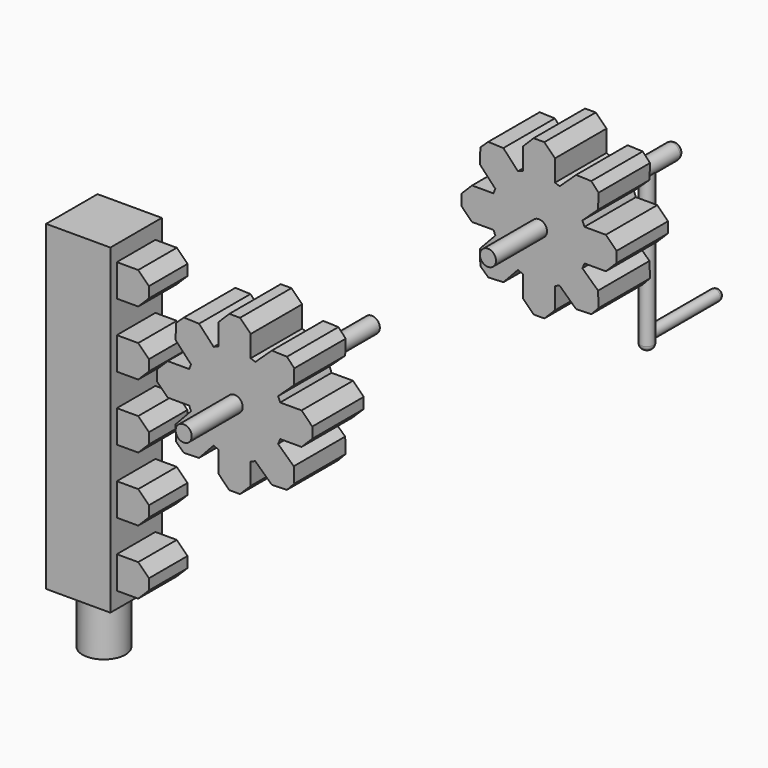
from build123d import *

# Parameters (mm, degrees)
F0_W           = 30.48
F0_H           = 30.48
F0_R           = 10.16
F1_DEPTH       = 152.4
F2_DEPTH       = 25.4
F3_W           = 22.86
F3_H           = 15.24
F4_DEPTH       = 30.48
F5_SIZE        = 5.08
F6_R           = 3.81
F7_DEPTH       = 30.48
F8_SIZE        = 5.08
F9_T1_DEPTH    = 56.6082991577
F9_T3_DEPTH    = 56.6285424882
F10_DEPTH      = 60.706
F10_DEPTH_BACK = 50.8
F13_R          = 3.1229358852
F14_DEPTH      = 76.2
F15_R          = 2.54
F17_R          = 2.667
F18_DEPTH      = 43.18
F19_R          = 2.54


# Not quite as in the source:
# - a fillet or chamfer that OpenCascade refuses, or shapes differently, is made with other operations: its cross-section is extruded or revolved along the edge and cut away or added


with BuildPart() as f1:
    # F0 (on Top) → F1 (new body)
    with BuildSketch(Plane.XY):
        Rectangle(F0_W, F0_H)
        Circle(F0_R, mode=Mode.SUBTRACT)
        Circle(F0_R)
    extrude(amount=F1_DEPTH)

    # F0 (on Top) → F2 (join)
    with BuildSketch(Plane.XY):
        Circle(F0_R)
    extrude(amount=-F2_DEPTH)

    # F3 (on Right) → F4 (join)
    with BuildSketch(Plane.YZ):
        with Locations((0, 15.24)):
            Rectangle(F3_W, F3_H)
        with Locations((0, 45.72)):
            Rectangle(F3_W, F3_H)
        with Locations((0, 76.2)):
            Rectangle(F3_W, F3_H)
        with Locations((0, 106.68)):
            Rectangle(F3_W, F3_H)
        with Locations((0, 137.16)):
            Rectangle(F3_W, F3_H)
    extrude(amount=F4_DEPTH)

    # F5
    f5_edges = [f1.edges().sort_by_distance(p)[0] for p in [
        (30.48, 0, 22.86),
        (30.48, 0, 7.62),
        (30.48, 0, 53.34),
        (30.48, 0, 38.1),
        (30.48, 0, 83.82),
        (30.48, 0, 68.58),
        (30.48, 0, 114.3),
        (30.48, 0, 99.06),
        (30.48, 0, 144.78),
        (30.48, 0, 129.54),
    ]]
    chamfer(f5_edges, length=F5_SIZE)


with BuildPart() as f7:
    # F6 (on Front) → F7 (new body)
    with BuildSketch(Plane.XZ):
        with BuildLine():
            ThreePointArc((107.9169317812, 108.821582713), (108.8951001643, 112.5759114794), (109.2243170907, 116.441582713))
            ThreePointArc((109.2243170907, 116.441582713), (108.8951001643, 120.3072539467), (107.9169317812, 124.061582713))
            ThreePointArc((107.9169317812, 124.061582713), (107.4603125366, 125.247181849), (106.9385318772, 126.405582207))
            ThreePointArc((106.9385318772, 126.405582207), (102.4405396502, 132.6938031218), (96.1037182714, 137.1230639134))
            ThreePointArc((96.1037182714, 137.1230639134), (95.0549396649, 137.5852030102), (93.9843170907, 137.9941974036))
            ThreePointArc((93.9843170907, 137.9941974036), (86.3643170907, 139.301582713), (78.7443170907, 137.9941974036))
            ThreePointArc((78.7443170907, 137.9941974036), (77.5587179546, 137.537578159), (76.4003175967, 137.0157974996))
            ThreePointArc((76.4003175967, 137.0157974996), (70.1120966819, 132.5178052726), (65.6828358903, 126.1809838937))
            ThreePointArc((65.6828358903, 126.1809838937), (65.209134246, 125.1040211001), (64.7914697966, 124.0041126884))
            ThreePointArc((64.7914697966, 124.0041126884), (63.5043983607, 116.3806265197), (64.8321074033, 108.7641126884))
            ThreePointArc((64.8321074033, 108.7641126884), (65.2323078484, 107.7227648238), (65.6828358903, 106.7021815323))
            ThreePointArc((65.6828358903, 106.7021815323), (70.1120966819, 100.3653601535), (76.4003175967, 95.8673679265))
            ThreePointArc((76.4003175967, 95.8673679265), (77.5587179546, 95.3455872671), (78.7443170907, 94.8889680225))
            ThreePointArc((78.7443170907, 94.8889680225), (86.3643170907, 93.581582713), (93.9843170907, 94.8889680225))
            ThreePointArc((93.9843170907, 94.8889680225), (95.0549396649, 95.2979624158), (96.1037182714, 95.7601015127))
            ThreePointArc((96.1037182714, 95.7601015127), (102.4405396502, 100.1893623043), (106.9385318772, 106.477583219))
            ThreePointArc((106.9385318772, 106.477583219), (107.4603125366, 107.635983577), (107.9169317812, 108.821582713))
        make_face()
        with Locations((86.3643170907, 116.441582713)):
            Circle(F6_R, mode=Mode.SUBTRACT)
        with BuildLine():
            ThreePointArc((78.7443170907, 137.9941974036), (86.3643170907, 139.301582713), (93.9843170907, 137.9941974036))
            Line((93.9843170907, 137.9941974036), (93.9843170907, 153.2341974036))
            Line((93.9843170907, 153.2341974036), (78.7443170907, 153.2341974036))
            Line((78.7443170907, 153.2341974036), (78.7443170907, 137.9941974036))
        make_face()
        with BuildLine():
            ThreePointArc((96.1037182714, 137.1230639134), (102.4405396502, 132.6938031218), (106.9385318772, 126.405582207))
            Line((106.9385318772, 126.405582207), (118.091235122, 136.7918621154))
            Line((118.091235122, 136.7918621154), (107.6959464169, 147.9361688564))
            Line((107.6959464169, 147.9361688564), (96.1037182714, 137.1230639134))
        make_face()
        with BuildLine():
            ThreePointArc((65.6828358903, 126.1809838937), (70.1120966819, 132.5178052726), (76.4003175967, 137.0157974996))
            Line((76.4003175967, 137.0157974996), (66.0140376883, 148.1685007444))
            Line((66.0140376883, 148.1685007444), (54.8697309473, 137.7732120393))
            Line((54.8697309473, 137.7732120393), (65.6828358903, 126.1809838937))
        make_face()
        with BuildLine():
            ThreePointArc((64.8321074033, 108.7641126884), (63.5043983607, 116.3806265197), (64.7914697966, 124.0041126884))
            Line((64.7914697966, 124.0041126884), (49.5514697966, 124.0041126884))
            Line((49.5514697966, 124.0041126884), (49.5514697966, 108.7641126884))
            Line((49.5514697966, 108.7641126884), (64.8321074033, 108.7641126884))
        make_face()
        with BuildLine():
            Line((66.0140376883, 84.7146646817), (76.4003175967, 95.8673679265))
            ThreePointArc((76.4003175967, 95.8673679265), (70.1120966819, 100.3653601535), (65.6828358903, 106.7021815323))
            Line((65.6828358903, 106.7021815323), (54.8697309473, 95.1099533868))
            Line((54.8697309473, 95.1099533868), (66.0140376883, 84.7146646817))
        make_face()
        with BuildLine():
            Line((93.9843170907, 79.6489680225), (93.9843170907, 94.8889680225))
            ThreePointArc((93.9843170907, 94.8889680225), (86.3643170907, 93.581582713), (78.7443170907, 94.8889680225))
            Line((78.7443170907, 94.8889680225), (78.7443170907, 79.6489680225))
            Line((78.7443170907, 79.6489680225), (93.9843170907, 79.6489680225))
        make_face()
        with BuildLine():
            ThreePointArc((107.9169317812, 124.061582713), (108.8951001643, 120.3072539467), (109.2243170907, 116.441582713))
            ThreePointArc((109.2243170907, 116.441582713), (108.8951001643, 112.5759114794), (107.9169317812, 108.821582713))
            Line((107.9169317812, 108.821582713), (123.1569317812, 108.821582713))
            Line((123.1569317812, 108.821582713), (123.1569317812, 124.061582713))
            Line((123.1569317812, 124.061582713), (107.9169317812, 124.061582713))
        make_face()
        with BuildLine():
            Line((118.091235122, 96.0913033107), (106.9385318772, 106.477583219))
            ThreePointArc((106.9385318772, 106.477583219), (102.4405396502, 100.1893623043), (96.1037182714, 95.7601015127))
            Line((96.1037182714, 95.7601015127), (107.6959464169, 84.9469965697))
            Line((107.6959464169, 84.9469965697), (118.091235122, 96.0913033107))
        make_face()
    extrude(amount=F7_DEPTH)

    # F8
    f8_edges = [f7.edges().sort_by_distance(p)[0] for p in [
        (78.744317, -15.24, 153.234197),
        (93.984317, -15.24, 153.234197),
    ]]
    chamfer(f8_edges, length=F8_SIZE)

    # F9: chamfer of 5.08 on 14 edges, made by hand

    # F9_s2 → F9_t1 (cut)
    with BuildSketch(Plane.XZ.offset(-13.0641495789)):
        Polygon((103.9811775033, 144.4710726214), (111.161042652, 144.2213999427), (107.6959464169, 147.9361688564), align=None)
        Polygon((118.0769317812, 124.061582713), (123.1569317812, 118.981582713), (123.1569317812, 124.061582713), align=None)
        Polygon((123.1569317812, 113.901582713), (118.0769317812, 108.821582713), (123.1569317812, 108.821582713), align=None)
        Polygon((111.161042652, 88.6617654833), (103.9811775033, 88.4120928047), (107.6959464169, 84.9469965697), align=None)
        Polygon((93.9843170907, 84.7289680225), (88.9043170907, 79.6489680225), (93.9843170907, 79.6489680225), align=None)
        Polygon((83.8243170907, 79.6489680225), (78.7443170907, 84.7289680225), (78.7443170907, 79.6489680225), align=None)
        Polygon((58.3348271823, 98.8247223004), (58.584499861, 91.6448571517), (54.8697309473, 95.1099533868), align=None)
        Polygon((54.6314697966, 124.0041126884), (49.5514697966, 118.9241126884), (49.5514697966, 124.0041126884), align=None)
        Polygon((49.5514697966, 113.8441126884), (54.6314697966, 108.7641126884), (49.5514697966, 108.7641126884), align=None)
        Polygon((58.584499861, 141.2383082743), (58.3348271823, 134.0584431256), (54.8697309473, 137.7732120393), align=None)
    extrude(amount=F9_T1_DEPTH, mode=Mode.SUBTRACT)

    # F9_s4 → F9_t3 (cut)
    with BuildSketch(Plane.XZ.offset(-13.0742712441)):
        Polygon((114.6233377073, 140.5096340438), (114.3706620964, 133.3269700605), (118.091235122, 136.7918621154), align=None)
        Polygon((114.3706620964, 99.5561953656), (114.6233377073, 92.3735313823), (118.091235122, 96.0913033107), align=None)
        Polygon((62.2962657599, 88.1825620964), (69.4789297432, 88.4352377073), (66.0140376883, 84.7146646817), align=None)
        Polygon((69.4789297432, 144.4479277188), (62.2962657599, 144.7006033297), (66.0140376883, 148.1685007444), align=None)
    extrude(amount=F9_T3_DEPTH, mode=Mode.SUBTRACT)

    # F6 (on Front) → F10 (join, two sides)
    with BuildSketch(Plane.XZ) as f10_sk:
        with Locations((86.3643170907, 116.441582713)):
            Circle(F6_R)
    extrude(amount=F10_DEPTH)
    extrude(f10_sk.sketch, amount=-F10_DEPTH_BACK)


with BuildPart() as f11_1:
    # F11: copy of F7
    add(f7.part.moved(Location((0, 180.34, 0))))

    # F13 (on offset) → F14 (join)
    with BuildSketch(Plane(origin=(0, 0, 116.441582713), x_dir=(1, 0, 0), z_dir=(0, 0, -1))):
        with Locations((86.4974185824, -213.6742174625)):
            Circle(F13_R)
    extrude(amount=F14_DEPTH)

    # F15
    f15_edges = [f11_1.edges().sort_by_distance(p)[0] for p in [
        (82.554317, 231.14, 116.441583),
        (83.374483, 213.674217, 40.241583),
    ]]
    fillet(f15_edges, radius=F15_R)

    # F17 (on offset) → F18 (join)
    with BuildSketch(Plane(origin=(0, 213.36, 0), x_dir=(-1, 0, 0), z_dir=(0, 1, 0))):
        with Locations((-86.4115506411, 46.1494922638)):
            Circle(F17_R)
    extrude(amount=F18_DEPTH)

    # F19
    f19_edges = [f11_1.edges().sort_by_distance(p)[0] for p in [
        (89.078551, 256.54, 46.149492),
    ]]
    fillet(f19_edges, radius=F19_R)


solid = Compound([f1.part, f7.part, f11_1.part])
